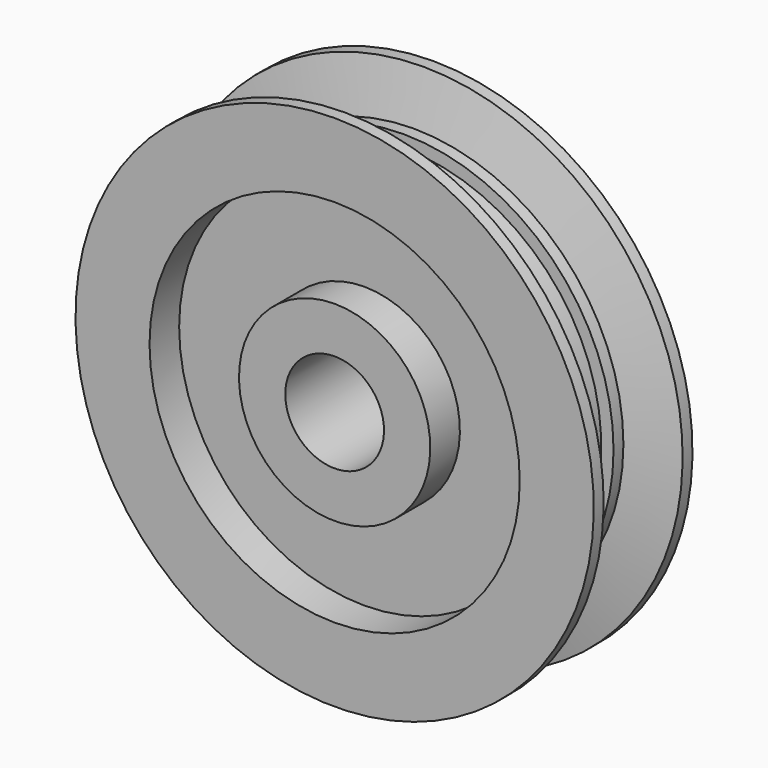
from build123d import *


# Not quite as in the source:
# - a feature names something its author has since deleted; it is built from what else it names


with BuildPart() as f1:
    # F0 (on Right) → F1 (revolve)
    with BuildSketch(Plane.YZ):
        Polygon((-23.5091740638, 16.747707203), (-23.5091740638, 19.747707203), (-24.0091740638, 19.747707203), (-24.5091740638, 17.747707203), (-25.0091740638, 17.747707203), (-25.0091740638, 17.247707203), (-27.0091740638, 17.247707203), (-27.0091740638, 17.747707203), (-27.5091740638, 17.747707203), (-28.0091740638, 19.747707203), (-28.5091740638, 19.747707203), (-28.5091740638, 16.747707203), (-27.0091740638, 16.747707203), (-27.0091740638, 13.122707203), (-28.5091740638, 13.122707203), (-28.5091740638, 11.247707203), (-26.0091740638, 11.247707203), (-23.5091740638, 11.247707203), (-23.5091740638, 13.122707203), (-25.0091740638, 13.122707203), (-25.0091740638, 16.747707203), align=None)
    revolve(axis=Axis((0, -33.8120413944, 9.247707203), (0, 1, 0)))


solid = f1.part
